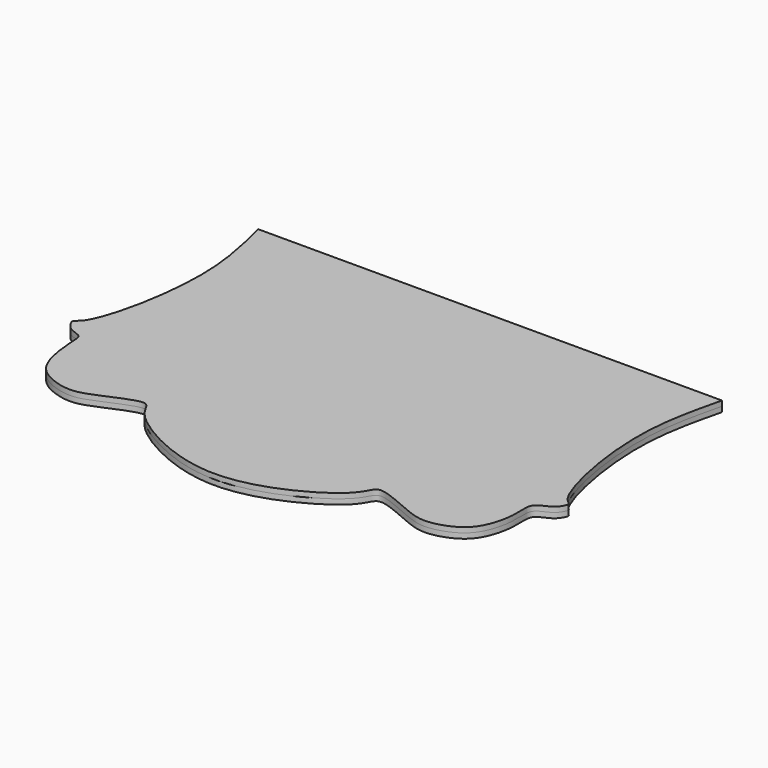
from build123d import *

# Parameters (mm, degrees)
F1_DEPTH = 2.5


with BuildPart() as f1:
    # F0 (on Top) → F1 (new body, symmetric)
    with BuildSketch(Plane.XY):
        with BuildLine():
            add(Edge.make_bspline(
                [(112.7518263381, -30), (110.0683866332, -41.2316047198), (101.557609718, -75.4725543916), (113.5357319655, -129.6037233134), (121.0880978452, -132.5225666296), (120.1512402386, -134.6893862512), (117.8203099052, -139.0537945373), (108.5063446408, -141.127301968), (110.834911802, -152.2990319153), (106.7349782851, -169.57347089), (96.1962562119, -176.1766582928), (85.6659613701, -178.4592822583), (76.5656283591, -175.7890482771), (58.4713403875, -167.0761326186), (55.2484363403, -169.6677039086), (53.716699705, -172.4040985511), (48.8397722553, -181.2039244379), (-9.3679e-06, -208.9860419393), (-48.839745919, -181.2039320243), (-53.716728711, -172.4040895936), (-55.2483775265, -169.6677221612), (-58.4717375728, -167.076009291), (-76.5620163803, -175.7901698806), (-85.6752558963, -178.4563960867), (-96.1609696724, -176.1876156046), (-106.8941817396, -169.5240344209), (-110.1818375624, -152.5018270408), (-110.1830537947, -142.1886320016), (-111.9097986439, -140.3301668428), (-117.8000702343, -138.8540242127), (-120.1728726925, -134.6810189597), (-121.0799907347, -132.525701525), (-113.5464604846, -129.5995892682), (-101.5562579572, -75.4725971802), (-110.0673297713, -41.2318534903), (-112.7511285434, -30)],
                knots=[0.5164160728, 0.5164160728, 0.5164160728, 0.5164160728, 0.5341655307, 0.5674378641, 0.5765384861, 0.5817683397, 0.5908163485, 0.6023499757, 0.6153069574, 0.6326235914, 0.6469289094, 0.6599795987, 0.6733921502, 0.6915691015, 0.6988100765, 0.7055701771, 0.7177536596, 0.7477870515, 0.7778204434, 0.7900039259, 0.7967640266, 0.8040050015, 0.8221819528, 0.8355945043, 0.8486451936, 0.8629505116, 0.8802671456, 0.8932241273, 0.8991974648, 0.9091836515, 0.9182316603, 0.9234615139, 0.9325621359, 0.9658344693, 0.9835842271, 0.9835842271, 0.9835842271, 0.9835842271], degree=3))
            Line((112.7518263381, -30), (-112.7511285434, -30))
        make_face()
    extrude(amount=F1_DEPTH, both=True)


solid = f1.part
